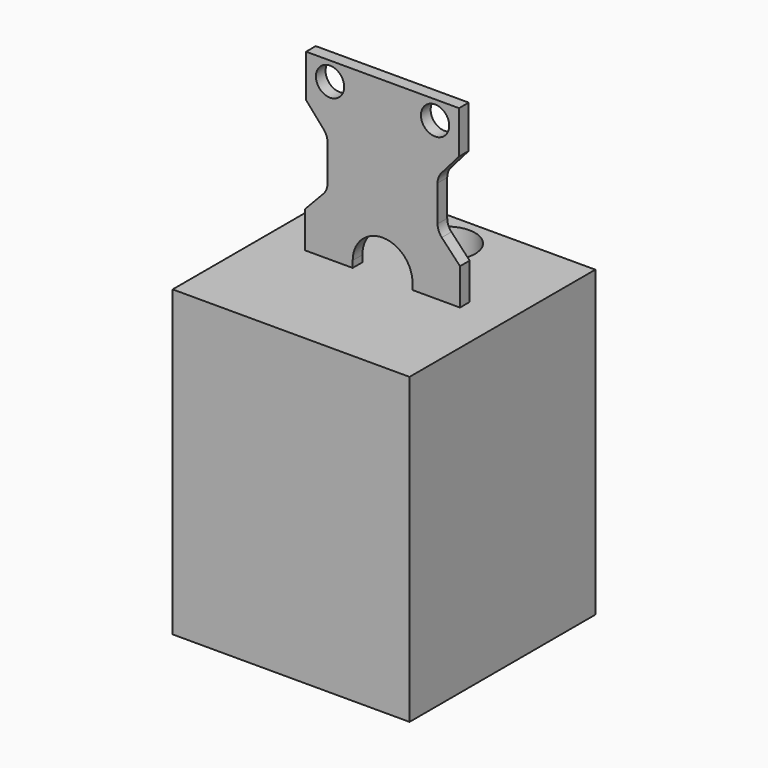
from build123d import *

# Parameters (mm, degrees)
F0_R          = 1.825
F1_DEPTH      = 1.56
F2_R          = 2
F3_R          = 0.5
F4_W          = 30.5997557007
F4_H          = 39.236785844
F5_DEPTH      = 15
F5_DEPTH_BACK = 15
F7_R          = 3.6749201005
F8_DEPTH      = 54.4


with BuildPart() as f1:
    # F0 (on Front) → F1 (new body)
    with BuildSketch(Plane.XZ):
        with BuildLine():
            Line((19.76, 0), (0, 0))
            Line((0, 0), (0, -5.5))
            Line((0, -5.5), (2.775, -8.679432))
            Line((2.775, -8.679432), (2.775, -14.859432))
            Line((2.775, -14.859432), (-0.12, -17.93))
            Line((-0.12, -17.93), (-0.12, -53.56))
            Line((-0.12, -53.56), (2.95, -57.14))
            Line((2.95, -57.14), (6.02, -53.56))
            Line((6.02, -53.56), (6.02, -21.79))
            ThreePointArc((6.02, -21.79), (9.88, -17.93), (13.74, -21.79))
            Line((13.74, -21.79), (13.74, -53.56))
            Line((13.74, -53.56), (16.81, -57.14))
            Line((16.81, -57.14), (19.88, -53.56))
            Line((19.88, -53.56), (19.88, -17.93))
            Line((19.88, -17.93), (16.985, -14.859432))
            Line((16.985, -14.859432), (16.985, -8.679432))
            Line((16.985, -8.679432), (19.76, -5.5))
            Line((19.76, -5.5), (19.76, 0))
        make_face()
        with Locations((3.095, -2.405)):
            Circle(F0_R, mode=Mode.SUBTRACT)
        with Locations((16.665, -2.405)):
            Circle(F0_R, mode=Mode.SUBTRACT)
    extrude(amount=F1_DEPTH)

    # F2
    f2_edges = [f1.edges().sort_by_distance(p)[0] for p in [
        (2.775, -0.78, -8.679432),
        (2.775, -0.78, -14.859432),
        (16.985, -0.78, -8.679432),
        (16.985, -0.78, -14.859432),
    ]]
    fillet(f2_edges, radius=F2_R)

    # F3
    f3_edges = [f1.edges().sort_by_distance(p)[0] for p in [
        (2.95, -0.78, -57.14),
        (16.81, -0.78, -57.14),
    ]]
    fillet(f3_edges, radius=F3_R)


with BuildPart() as f5:
    # F4 (on face) → F5 (new body, two sides)
    with BuildSketch(Plane.XZ.offset(1.56)) as f5_sk:
        with Locations((10.0650798995, -42.2559035942)):
            Rectangle(F4_W, F4_H)
    extrude(amount=-F5_DEPTH)
    extrude(f5_sk.sketch, amount=F5_DEPTH_BACK)

    # F6: cut F1
    add(f1.part, mode=Mode.SUBTRACT)

    # F7 (on face) → F8 (cut)
    with BuildSketch(Plane.XY.offset(-22.6375106722)):
        with Locations((10.0650798995, 8.5569592193)):
            Circle(F7_R)
    extrude(amount=-F8_DEPTH, mode=Mode.SUBTRACT)


solid = Compound([f1.part, f5.part])
